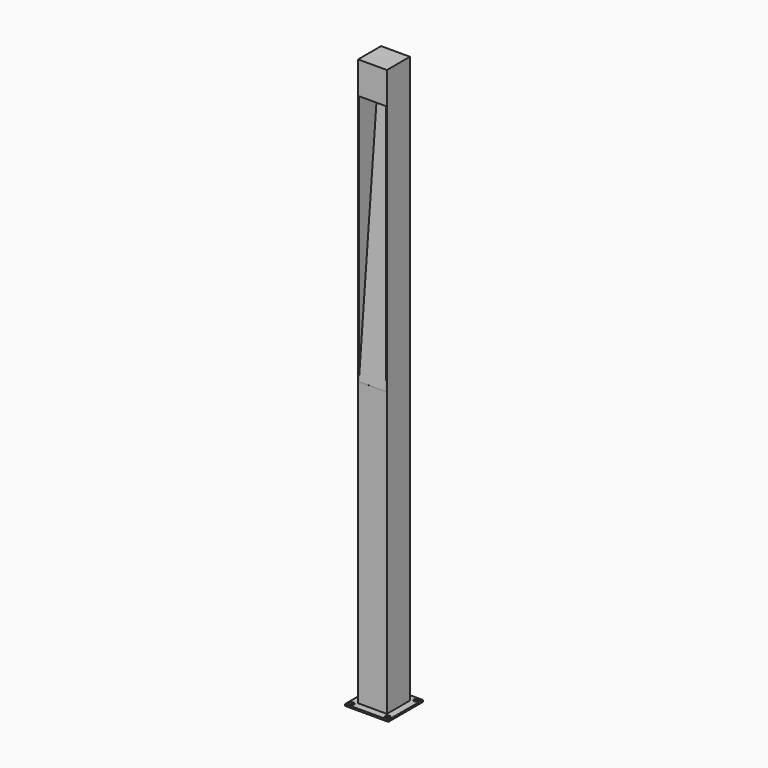
from build123d import *

# Parameters (mm, degrees)
F0_W      = 50.8
F0_H      = 25.4
F0_W_2    = 47
F0_H_2    = 21.6
F1_DEPTH  = 1500
F2_W      = 228.6
F2_H      = 228.6
F2_R      = 12.7
F3_DEPTH  = 9.525
F4_W      = 144.553527236
F4_H      = 1330
F5_DEPTH  = 81
F6_W      = 152.4
F6_H      = 152.4
F7_DEPTH  = 1.9
F9_DEPTH  = 72.2
F10_R     = 12.7
F11_DEPTH = 1.9


# Not quite as in the source:
# - a length typed as a fraction of an inch, garbled in the dataset ("3 / 203.2 mm" for 3/8 in), is restored


with BuildPart() as f1:
    # F0 (on Top) → F1 (new body, symmetric)
    with BuildSketch(Plane.XY):
        with Locations((0, -63.5)):
            Rectangle(F0_W, F0_H)
        with Locations((0, -63.5)):
            Rectangle(F0_W_2, F0_H_2, mode=Mode.SUBTRACT)
        with Locations((0, 63.5)):
            Rectangle(F0_W, F0_H)
        with Locations((0, 63.5)):
            Rectangle(F0_W_2, F0_H_2, mode=Mode.SUBTRACT)
        Polygon((-25.4, 76.2), (-76.2, 76.2), (-76.2, -76.2), (-25.4, -76.2), (-25.4, -50.8), (-27.3, -50.8), (-27.3, -74.3), (-74.3, -74.3), (-74.3, 74.3), (-27.3, 74.3), (-27.3, 50.8), (-25.4, 50.8), align=None)
        Polygon((76.2, 76.2), (25.4, 76.2), (25.4, 50.8), (27.3, 50.8), (27.3, 74.3), (74.3, 74.3), (74.3, -74.3), (27.3, -74.3), (27.3, -50.8), (25.4, -50.8), (25.4, -76.2), (76.2, -76.2), align=None)
    extrude(amount=F1_DEPTH, both=True)

    # F4 (on face) → F5 (cut)
    with BuildSketch(Plane.XZ.offset(76.2)):
        with Locations((0, 665)):
            Rectangle(F4_W, F4_H)
    extrude(amount=-F5_DEPTH, mode=Mode.SUBTRACT)

    # F6 (on face) → F7 (join)
    with BuildSketch(Plane.XY.offset(1500)):
        Rectangle(F6_W, F6_H)
    extrude(amount=-F7_DEPTH)

    # F8 (on Right) → F9 (join, symmetric)
    with BuildSketch(Plane.YZ):
        Polygon((-76.1449276874, 0.0104757039), (-74.2529536564, -0.1639841968), (50.611830749, 1343.0530421202), (48.719856718, 1343.2275020208), align=None)
    extrude(amount=F9_DEPTH, both=True)

    # F10 (on face) → F11 (cut, through all)
    with BuildSketch(Plane.XZ.offset(-50.8)):
        with Locations((0, 1448.3414888382)):
            Circle(F10_R)
    extrude(amount=-F11_DEPTH, mode=Mode.SUBTRACT)


with BuildPart() as f3:
    # F2 (on face) → F3 (new body)
    with BuildSketch(Plane(origin=(0, 0, -1500), x_dir=(1, 0, 0), z_dir=(0, 0, -1))):
        Rectangle(F2_W, F2_H)
        with Locations((-95.25, -95.25)):
            Circle(F2_R, mode=Mode.SUBTRACT)
        with Locations((95.25, -95.25)):
            Circle(F2_R, mode=Mode.SUBTRACT)
        with Locations((-95.25, 95.25)):
            Circle(F2_R, mode=Mode.SUBTRACT)
        Circle(F2_R, mode=Mode.SUBTRACT)
        with Locations((95.25, 95.25)):
            Circle(F2_R, mode=Mode.SUBTRACT)
    extrude(amount=F3_DEPTH)


solid = Compound([f1.part, f3.part])
